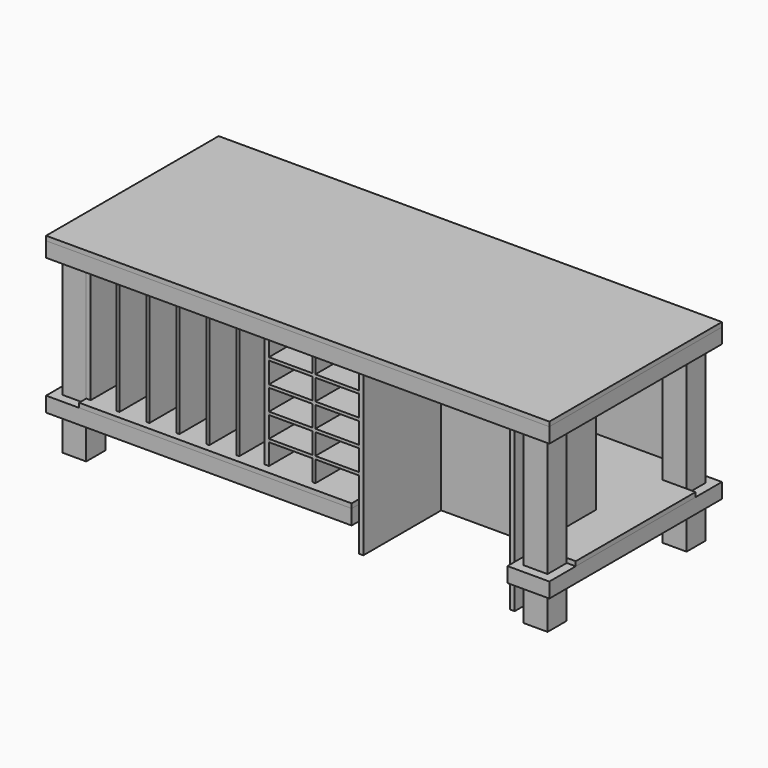
from build123d import *

# Parameters (mm, degrees)
F0_W           = 2133.6
F0_H           = 914.4
F1_DEPTH       = 19.05
F2_W           = 38.1
F2_H           = 838.2
F3_DEPTH       = 63.5
F4_W           = 101.6
F4_H           = 101.6
F5_DEPTH       = 793.75
F7_W           = 101.6
F7_H           = 38.1
F7_W_2         = 38.1
F7_H_2         = 838.2
F7_H_3         = 368.3
F8_DEPTH       = 63.5
F10_DEPTH      = 19.05
F11_W          = 622.3
F11_H          = 19.05
F12_DEPTH      = 495.3
F12_DEPTH_BACK = 203.2
F14_DEPTH      = 495.3
F15_W          = 12.7
F15_H          = 482.6
F15_H_2        = 12.7
F16_DEPTH      = 863.6
F17_W          = 12.7
F17_H          = 88.9
F17_W_2        = 184.15
F17_H_2        = 12.7
F18_DEPTH      = 412.75


# Not quite as in the source:
# - a feature names something its author has since deleted; it is built from what else it names


with BuildPart() as f1:
    # F0 (on Top) → F1 (new body)
    with BuildSketch(Plane.XY):
        with Locations((1066.8, -457.2)):
            Rectangle(F0_W, F0_H)
    extrude(amount=-F1_DEPTH)


with BuildPart() as f3:
    # F2 (on face) → F3 (new body)
    with BuildSketch(Plane(origin=(0, 0, -19.05), x_dir=(1, 0, 0), z_dir=(0, 0, -1))):
        Polygon((38.1, 914.4), (0, 914.4), (0, 0), (38.1, 0), (38.1, 38.1), (38.1, 876.3), align=None)
        Polygon((2095.5, 914.4), (38.1, 914.4), (38.1, 876.3), (209.55, 876.3), (247.65, 876.3), (419.1, 876.3), (457.2, 876.3), (628.65, 876.3), (666.75, 876.3), (838.2, 876.3), (876.3, 876.3), (1047.75, 876.3), (1085.85, 876.3), (1257.3, 876.3), (1295.4, 876.3), (1466.85, 876.3), (1504.95, 876.3), (1676.4, 876.3), (1714.5, 876.3), (1885.95, 876.3), (1924.05, 876.3), (2095.5, 876.3), align=None)
        Polygon((2133.6, 914.4), (2095.5, 914.4), (2095.5, 876.3), (2095.5, 38.1), (2095.5, 0), (2133.6, 0), align=None)
        Polygon((38.1, 38.1), (38.1, 0), (2095.5, 0), (2095.5, 38.1), (1924.05, 38.1), (1885.95, 38.1), (1714.5, 38.1), (1676.4, 38.1), (1504.95, 38.1), (1466.85, 38.1), (1295.4, 38.1), (1257.3, 38.1), (1085.85, 38.1), (1047.75, 38.1), (876.3, 38.1), (838.2, 38.1), (666.75, 38.1), (628.65, 38.1), (457.2, 38.1), (419.1, 38.1), (247.65, 38.1), (209.55, 38.1), align=None)
        with Locations((228.6, 457.2)):
            Rectangle(F2_W, F2_H)
        with Locations((438.15, 457.2)):
            Rectangle(F2_W, F2_H)
        with Locations((647.7, 457.2)):
            Rectangle(F2_W, F2_H)
        with Locations((857.25, 457.2)):
            Rectangle(F2_W, F2_H)
        with Locations((1066.8, 457.2)):
            Rectangle(F2_W, F2_H)
        with Locations((1276.35, 457.2)):
            Rectangle(F2_W, F2_H)
        with Locations((1485.9, 457.2)):
            Rectangle(F2_W, F2_H)
        with Locations((1695.45, 457.2)):
            Rectangle(F2_W, F2_H)
        with Locations((1905, 457.2)):
            Rectangle(F2_W, F2_H)
    extrude(amount=F3_DEPTH)


with BuildPart() as f5:
    # F4 (on face) → F5 (new body)
    with BuildSketch(Plane(origin=(0, 0, -19.05), x_dir=(1, 0, 0), z_dir=(0, 0, -1))):
        with Locations((88.9, 825.5)):
            Rectangle(F4_W, F4_H)
    extrude(amount=F5_DEPTH)


with BuildPart() as f5b:
    # F4 (on face) → F5, piece 2 (new body)
    with BuildSketch(Plane(origin=(0, 0, -19.05), x_dir=(1, 0, 0), z_dir=(0, 0, -1))):
        with Locations((2044.7, 825.5)):
            Rectangle(F4_W, F4_H)
    extrude(amount=F5_DEPTH)


with BuildPart() as f5c:
    # F4 (on face) → F5, piece 3 (new body)
    with BuildSketch(Plane(origin=(0, 0, -19.05), x_dir=(1, 0, 0), z_dir=(0, 0, -1))):
        with Locations((88.9, 88.9)):
            Rectangle(F4_W, F4_H)
    extrude(amount=F5_DEPTH)


with BuildPart() as f5d:
    # F4 (on face) → F5, piece 4 (new body)
    with BuildSketch(Plane(origin=(0, 0, -19.05), x_dir=(1, 0, 0), z_dir=(0, 0, -1))):
        with Locations((2044.7, 88.9)):
            Rectangle(F4_W, F4_H)
    extrude(amount=F5_DEPTH)


with BuildPart() as f8:
    # F7 (on offset) → F8 (new body)
    with BuildSketch(Plane(origin=(0, 0, -660.4), x_dir=(1, 0, 0), z_dir=(0, 0, -1))):
        Polygon((38.1, 914.4), (0, 914.4), (0, 0), (38.1, 0), (38.1, 38.1), (38.1, 876.3), align=None)
        Polygon((1295.4, 914.4), (38.1, 914.4), (38.1, 876.3), (209.55, 876.3), (247.65, 876.3), (419.1, 876.3), (457.2, 876.3), (628.65, 876.3), (666.75, 876.3), (838.2, 876.3), (876.3, 876.3), (1047.75, 876.3), (1085.85, 876.3), (1257.3, 876.3), (1295.4, 876.3), align=None)
        Polygon((38.1, 38.1), (38.1, 0), (2095.5, 0), (2095.5, 38.1), (1924.05, 38.1), (1885.95, 38.1), (1714.5, 38.1), (1676.4, 38.1), (1504.95, 38.1), (1466.85, 38.1), (1295.4, 38.1), (1257.3, 38.1), (1085.85, 38.1), (1047.75, 38.1), (876.3, 38.1), (838.2, 38.1), (666.75, 38.1), (628.65, 38.1), (457.2, 38.1), (419.1, 38.1), (247.65, 38.1), (209.55, 38.1), align=None)
        Polygon((1295.4, 444.5), (1295.4, 876.3), (1257.3, 876.3), (1257.3, 38.1), (1295.4, 38.1), (1295.4, 406.4), align=None)
        Polygon((2095.5, 38.1), (2095.5, 0), (2133.6, 0), (2133.6, 914.4), (2095.5, 914.4), (2095.5, 876.3), (2095.5, 444.5), (2095.5, 406.4), align=None)
        Polygon((1955.8, 444.5), (1295.4, 444.5), (1295.4, 406.4), (1466.85, 406.4), (1504.95, 406.4), (1676.4, 406.4), (1714.5, 406.4), (1885.95, 406.4), (1924.05, 406.4), (2095.5, 406.4), (2095.5, 444.5), (1993.9, 444.5), align=None)
        Polygon((1955.8, 914.4), (1955.8, 444.5), (1993.9, 444.5), (1993.9, 876.3), (1993.9, 914.4), align=None)
        with Locations((2044.7, 895.35)):
            Rectangle(F7_W, F7_H)
        with Locations((228.6, 457.2)):
            Rectangle(F7_W_2, F7_H_2)
        with Locations((438.15, 457.2)):
            Rectangle(F7_W_2, F7_H_2)
        with Locations((647.7, 457.2)):
            Rectangle(F7_W_2, F7_H_2)
        with Locations((857.25, 457.2)):
            Rectangle(F7_W_2, F7_H_2)
        with Locations((1066.8, 457.2)):
            Rectangle(F7_W_2, F7_H_2)
        with Locations((1485.9, 222.25)):
            Rectangle(F7_W_2, F7_H_3)
        with Locations((1695.45, 222.25)):
            Rectangle(F7_W_2, F7_H_3)
        with Locations((1905, 222.25)):
            Rectangle(F7_W_2, F7_H_3)
    extrude(amount=-F8_DEPTH)


with BuildPart() as f10:
    # F9 (on face) → F10 (new body)
    with BuildSketch(Plane.XY.offset(-596.9)):
        Polygon((139.7, -139.7), (0, -139.7), (0, -774.7), (139.7, -774.7), (139.7, -914.4), (1295.4, -914.4), (1295.4, -444.5), (1955.8, -444.5), (1955.8, -774.7), (1993.9, -774.7), (2133.6, -774.7), (2133.6, -139.7), (1993.9, -139.7), (1993.9, 0), (139.7, 0), align=None)
    extrude(amount=F10_DEPTH)


with BuildPart() as f12:
    # F11 (on face) → F12 (new body, two sides)
    with BuildSketch(Plane.XY.offset(-577.85)) as f12_sk:
        Polygon((1314.45, -444.5), (1295.4, -444.5), (1295.4, -876.3), (1314.45, -876.3), (1314.45, -463.55), align=None)
        with Locations((1625.6, -454.025)):
            Rectangle(F11_W, F11_H)
        Polygon((1955.8, -444.5), (1936.75, -444.5), (1936.75, -463.55), (1936.75, -876.3), (1955.8, -876.3), (1955.8, -774.7), align=None)
    extrude(amount=F12_DEPTH)
    extrude(f12_sk.sketch, amount=-F12_DEPTH_BACK)


with BuildPart() as f14:
    # F13 (on face) → F14 (new body)
    with BuildSketch(Plane.XY.offset(-577.85)):
        Polygon((158.75, -19.05), (139.7, -19.05), (139.7, -139.7), (139.7, -774.7), (139.7, -876.3), (158.75, -876.3), align=None)
        Polygon((1993.9, 0), (139.7, 0), (139.7, -19.05), (158.75, -19.05), (895.35, -19.05), (895.35, -444.5), (895.35, -876.3), (914.4, -876.3), (914.4, -463.55), (1295.4, -463.55), (1295.4, -444.5), (914.4, -444.5), (914.4, -19.05), (1993.9, -19.05), align=None)
    extrude(amount=F14_DEPTH)


with BuildPart() as f16:
    # F15 (on face) → F16 (new body)
    with BuildSketch(Plane.XZ.offset(19.05)):
        with Locations((406.4, -336.55)):
            Rectangle(F15_W, F15_H)
        with Locations((406.4, -88.9)):
            Rectangle(F15_W, F15_H_2)
    extrude(amount=F16_DEPTH)


with BuildPart() as f16b:
    # F15 (on face) → F16, piece 2 (new body)
    with BuildSketch(Plane.XZ.offset(19.05)):
        with Locations((279.4, -336.55)):
            Rectangle(F15_W, F15_H)
    extrude(amount=F16_DEPTH)


with BuildPart() as f16c:
    # F15 (on face) → F16, piece 3 (new body)
    with BuildSketch(Plane.XZ.offset(19.05)):
        with Locations((533.4, -336.55)):
            Rectangle(F15_W, F15_H)
        with Locations((533.4, -88.9)):
            Rectangle(F15_W, F15_H_2)
    extrude(amount=F16_DEPTH)


with BuildPart() as f16d:
    # F15 (on face) → F16, piece 4 (new body)
    with BuildSketch(Plane.XZ.offset(19.05)):
        with Locations((660.4, -336.55)):
            Rectangle(F15_W, F15_H)
        with Locations((660.4, -88.9)):
            Rectangle(F15_W, F15_H_2)
    extrude(amount=F16_DEPTH)


with BuildPart() as f16e:
    # F15 (on face) → F16, piece 5 (new body)
    with BuildSketch(Plane.XZ.offset(19.05)):
        with Locations((787.4, -336.55)):
            Rectangle(F15_W, F15_H)
        with Locations((787.4, -88.9)):
            Rectangle(F15_W, F15_H_2)
    extrude(amount=F16_DEPTH)


with BuildPart() as f18:
    # F17 (on face) → F18 (new body)
    with BuildSketch(Plane.XZ.offset(463.55)):
        with Locations((1104.9, -127)):
            Rectangle(F17_W, F17_H)
        with Locations((1006.475, -177.8)):
            Rectangle(F17_W_2, F17_H_2)
        with Locations((1104.9, -177.8)):
            Rectangle(F17_W, F17_H_2)
        with Locations((1203.325, -177.8)):
            Rectangle(F17_W_2, F17_H_2)
        with Locations((1104.9, -228.6)):
            Rectangle(F17_W, F17_H)
        with Locations((1006.475, -279.4)):
            Rectangle(F17_W_2, F17_H_2)
        with Locations((1104.9, -279.4)):
            Rectangle(F17_W, F17_H_2)
        with Locations((1203.325, -279.4)):
            Rectangle(F17_W_2, F17_H_2)
        with Locations((1104.9, -330.2)):
            Rectangle(F17_W, F17_H)
        with Locations((1006.475, -381)):
            Rectangle(F17_W_2, F17_H_2)
        with Locations((1104.9, -381)):
            Rectangle(F17_W, F17_H_2)
        with Locations((1203.325, -381)):
            Rectangle(F17_W_2, F17_H_2)
        with Locations((1104.9, -431.8)):
            Rectangle(F17_W, F17_H)
        with Locations((1006.475, -482.6)):
            Rectangle(F17_W_2, F17_H_2)
        with Locations((1104.9, -482.6)):
            Rectangle(F17_W, F17_H_2)
        with Locations((1203.325, -482.6)):
            Rectangle(F17_W_2, F17_H_2)
        with Locations((1104.9, -533.4)):
            Rectangle(F17_W, F17_H)
    extrude(amount=F18_DEPTH)


solid = Compound([f1.part, f3.part, f5.part, f5b.part, f5c.part, f5d.part, f8.part, f10.part, f12.part, f14.part, f16.part, f16b.part, f16c.part, f16d.part, f16e.part, f18.part])
